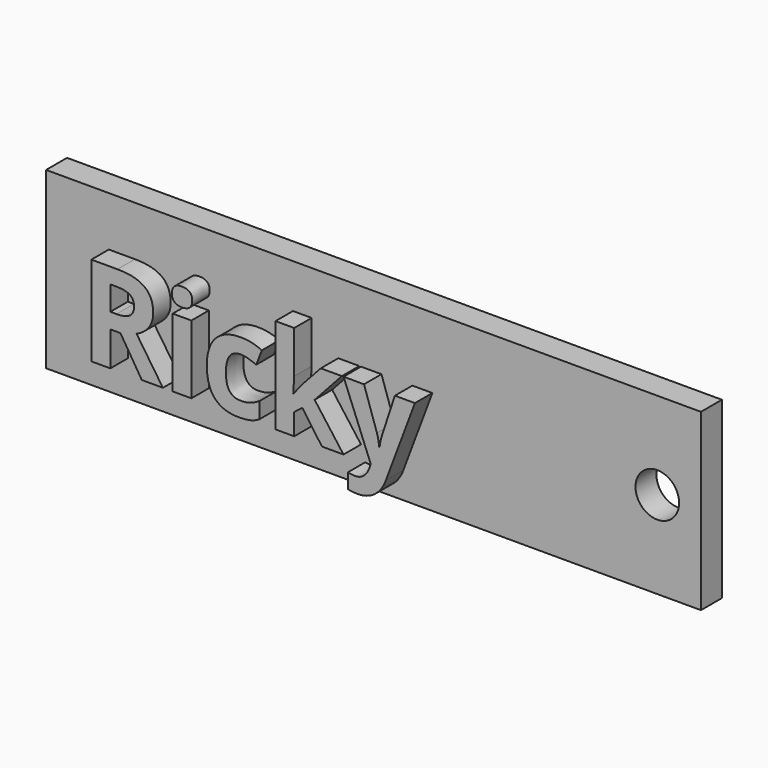
from build123d import *

# Parameters (mm, degrees)
F0_W         = 75
F0_H         = 20
F0_R         = 2.5
F1_DEPTH     = 3
F2_TEXT_SIZE = 14.3704379702
F3_DEPTH     = 2.5


# Not quite as in the source:
# - Text() gives the source's letters only with a copy of the font that has no kerning and outlines rounded to 1/6400 em; it was checked with that copy


with BuildPart() as f1:
    # F0 (on Front) → F1 (new body)
    with BuildSketch(Plane.XZ):
        with Locations((37.5, -10)):
            Rectangle(F0_W, F0_H)
        with Locations((70, -10)):
            Circle(F0_R, mode=Mode.SUBTRACT)
    extrude(amount=F1_DEPTH)

    # F2 (on face) → F3 (join)
    with BuildSketch(Plane.XZ.offset(3)):
        with Locations((5.8918814175, -15.9511864185)):
            Text('Ricky', F2_TEXT_SIZE, font='Open Sans', font_style=FontStyle.BOLD, text_align=(TextAlign.LEFT, TextAlign.BOTTOM))
    extrude(amount=F3_DEPTH)


solid = f1.part
